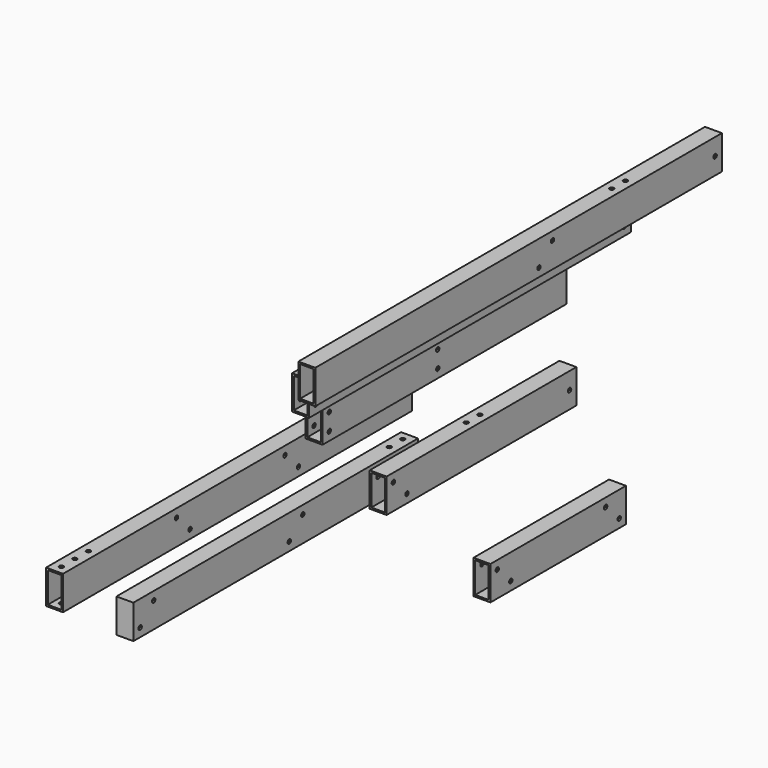
from build123d import *

# Parameters (mm, degrees)
F0_W      = 25.4
F0_H      = 50.8
F1_DEPTH  = 177.8
F2_T      = -2.54
F3_W      = 25.4
F3_H      = 50.8
F4_DEPTH  = 301.625
F5_T      = -2.54
F6_W      = 25.4
F6_H      = 50.8
F7_DEPTH  = 228.6
F8_T      = -2.54
F9_R      = 3.175
F10_DEPTH = 80.8299855063
F11_R     = 3.175
F12_DEPTH = 50.801
F13_R     = 3.175
F14_DEPTH = 63.5847636232
F15_R     = 3.175
F16_DEPTH = 223.7081707755
F17_R     = 3.175
F18_DEPTH = 25.401
F19_R     = 3.175
F20_DEPTH = 128.3850575145
F21_W     = 25.4
F21_H     = 50.8
F22_DEPTH = 381
F23_T     = -2.54
F24_R     = 3.175
F25_DEPTH = 136.5013085971
F26_R     = 3.175
F27_DEPTH = 295.0848142092
F28_W     = 25.4
F28_H     = 50.8
F29_DEPTH = 127
F30_T     = -2.54
F31_R     = 3.175
F32_DEPTH = 195.8388724098
F33_W     = 25.4
F33_H     = 50.8
F34_DEPTH = 533.4
F35_T     = -2.54
F36_W     = 25.4
F36_H     = 50.8
F37_DEPTH = 654.05
F38_T     = -2.54
F40_D     = 6.35
F40_DEPTH = 50.8
F40_TIP   = 1.9077324654
F42_D     = 6.35
F42_DEPTH = 50.8
F42_TIP   = 1.9077324654
F44_D     = 6.35
F44_DEPTH = 50.8
F44_TIP   = 1.9077324654
F47_D     = 6.35
F47_DEPTH = 50.8
F47_TIP   = 1.9077324654
F49_D     = 6.35
F49_DEPTH = 50.8
F49_TIP   = 1.9077324654
F50_D     = 6.35
F50_DEPTH = 50.8
F50_TIP   = 1.9077324654
F51_D     = 6.35
F51_DEPTH = 50.8
F51_TIP   = 1.9077324654
F52_D     = 6.35
F52_DEPTH = 50.8
F52_TIP   = 1.9077324654


# Not quite as in the source:
# - a pattern or mirror of a feature is missing from the dataset's text; its kind, count and spacing are read off the source's solid


with BuildPart() as f1:
    # F0 (on Front) → F1 (new body, symmetric)
    with BuildSketch(Plane.XZ):
        with Locations((17.2452218831, 6.8087904424)):
            Rectangle(F0_W, F0_H)
    extrude(amount=F1_DEPTH, both=True)

    # F2
    f2_openings = [f1.faces().sort_by_distance(p)[0] for p in [
        (17.245222, -177.8, 6.80879),
        (17.245222, 177.8, 6.80879),
    ]]
    offset(amount=F2_T, openings=f2_openings)

    # F9 (on face) → F10 (cut, through all)
    with BuildSketch(Plane.YZ.offset(29.9452218831)):
        with Locations((-165.1, 19.5087904424)):
            Circle(F9_R)
        with Locations((-139.7, -5.8912095576)):
            Circle(F9_R)
        with Locations((165.1, 6.8087904424)):
            Circle(F9_R)
    extrude(amount=-F10_DEPTH, mode=Mode.SUBTRACT)

    # F11 (on face) → F12 (cut, through all)
    with BuildSketch(Plane.XY.offset(32.2087904424)):
        with Locations((17.2452218831, 12.7)):
            Circle(F11_R)
        with Locations((17.2452218831, -12.7)):
            Circle(F11_R)
    extrude(amount=-F12_DEPTH, mode=Mode.SUBTRACT)


with BuildPart() as f4:
    # F3 (on Front) → F4 (new body, symmetric)
    with BuildSketch(Plane.XZ):
        with Locations((0, 179.7159612179)):
            Rectangle(F3_W, F3_H)
    extrude(amount=F4_DEPTH, both=True)

    # F5
    f5_openings = [f4.faces().sort_by_distance(p)[0] for p in [
        (0, -301.625, 179.715961),
        (0, 301.625, 179.715961),
    ]]
    offset(amount=F5_T, openings=f5_openings)

    # F13 (on face) → F14 (cut, through all)
    with BuildSketch(Plane.YZ.offset(12.7)):
        with Locations((-288.925, 192.4159612179)):
            Circle(F13_R)
        with Locations((-288.925, 167.0159612179)):
            Circle(F13_R)
    f14 = extrude(amount=-F14_DEPTH, mode=Mode.SUBTRACT)

    # F14_copies: F14 across plane
    add(f14.mirror(Plane.ZX), mode=Mode.SUBTRACT)

    # F15 (on face) → F16 (cut, through all)
    with BuildSketch(Plane.XY.offset(205.1159612179)):
        with Locations((0, -114.3)):
            Circle(F15_R)
        with Locations((0, -88.9)):
            Circle(F15_R)
    f16 = extrude(amount=-F16_DEPTH, mode=Mode.SUBTRACT)

    # F16_copies: F16 across plane
    add(f16.mirror(Plane.ZX), mode=Mode.SUBTRACT)


with BuildPart() as f7:
    # F6 (on Front) → F7 (new body, symmetric)
    with BuildSketch(Plane.XZ):
        with Locations((-38.1837636232, 102.1319037034)):
            Rectangle(F6_W, F6_H)
    extrude(amount=F7_DEPTH, both=True)

    # F8
    f8_openings = [f7.faces().sort_by_distance(p)[0] for p in [
        (-38.183764, -228.6, 102.131904),
        (-38.183764, 228.6, 102.131904),
    ]]
    offset(amount=F8_T, openings=f8_openings)

    # F17 (on face) → F18 (cut, through all)
    with BuildSketch(Plane.YZ.offset(-25.4837636232)):
        with Locations((-215.9, 114.8319037034)):
            Circle(F17_R)
        with Locations((-215.9, 89.4319037034)):
            Circle(F17_R)
        with Locations((-12.7, 114.8319037034)):
            Circle(F17_R)
        with Locations((-12.7, 89.4319037034)):
            Circle(F17_R)
    extrude(amount=-F18_DEPTH, mode=Mode.SUBTRACT)

    # F19 (on face) → F20 (cut, through all)
    with BuildSketch(Plane(origin=(0, 0, 76.7319037034), x_dir=(1, 0, 0), z_dir=(0, 0, -1))):
        with Locations((-38.1837636232, -215.9)):
            Circle(F19_R)
        with Locations((-38.1837636232, -190.5)):
            Circle(F19_R)
    extrude(amount=-F20_DEPTH, mode=Mode.SUBTRACT)


with BuildPart() as f22:
    # F21 (on Front) → F22 (new body, symmetric)
    with BuildSketch(Plane.XZ):
        with Locations((72.9165449739, 251.0926046515)):
            Rectangle(F21_W, F21_H)
    extrude(amount=F22_DEPTH, both=True)

    # F23
    f23_openings = [f22.faces().sort_by_distance(p)[0] for p in [
        (72.916545, -381, 251.092605),
        (72.916545, 381, 251.092605),
    ]]
    offset(amount=F23_T, openings=f23_openings)

    # F24 (on face) → F25 (cut, through all)
    with BuildSketch(Plane.YZ.offset(85.6165449739)):
        with Locations((368.3, 251.0926046515)):
            Circle(F24_R)
        with Locations((63.5, 263.7926046515)):
            Circle(F24_R)
        with Locations((38.1, 238.3926046515)):
            Circle(F24_R)
    extrude(amount=-F25_DEPTH, mode=Mode.SUBTRACT)

    # F26 (on face) → F27 (cut, through all)
    with BuildSketch(Plane.XY.offset(276.4926046515)):
        with Locations((72.9165449739, 215.9)):
            Circle(F26_R)
        with Locations((72.9165449739, 190.5)):
            Circle(F26_R)
    extrude(amount=-F27_DEPTH, mode=Mode.SUBTRACT)


with BuildPart() as f29:
    # F28 (on Front) → F29 (new body, symmetric)
    with BuildSketch(Plane.XZ):
        with Locations((132.2541087866, -91.8391663149)):
            Rectangle(F28_W, F28_H)
    extrude(amount=F29_DEPTH, both=True)

    # F30
    f30_openings = [f29.faces().sort_by_distance(p)[0] for p in [
        (132.254109, -127, -91.839166),
        (132.254109, 127, -91.839166),
    ]]
    offset(amount=F30_T, openings=f30_openings)

    # F31 (on face) → F32 (cut, through all)
    with BuildSketch(Plane.YZ.offset(144.9541087866)):
        with Locations((-114.3, -79.1391663149)):
            Circle(F31_R)
        with Locations((-88.9, -104.5391663149)):
            Circle(F31_R)
        with Locations((88.9, -79.1391663149)):
            Circle(F31_R)
        with Locations((114.3, -104.5391663149)):
            Circle(F31_R)
    extrude(amount=-F32_DEPTH, mode=Mode.SUBTRACT)


with BuildPart() as f34:
    # F33 (on Front) → F34 (new body)
    with BuildSketch(Plane.XZ):
        with Locations((-77.9336839914, -46.0702102427)):
            Rectangle(F33_W, F33_H)
    extrude(amount=F34_DEPTH)

    # F35
    f35_openings = [f34.faces().sort_by_distance(p)[0] for p in [
        (-77.933684, 0, -46.07021),
    ]]
    offset(amount=F35_T, openings=f35_openings)

    # F42
    with Locations(Plane(origin=(0, 0, -71.4702102427), x_dir=(1, 0, 0), z_dir=(0, 0, -1))):
        with Locations((-77.9336839914, 12.7), (-77.9336839914, 38.1)):
            Hole(F42_D / 2, depth=F42_DEPTH)
            with Locations((0, 0, -(F42_DEPTH + F42_TIP / 2))):  # 118° drill point
                Cone(0, F42_D / 2, F42_TIP, mode=Mode.SUBTRACT)

    # F47
    with Locations(Plane(origin=(-90.6336839914, 0, 0), x_dir=(0, -1, 0), z_dir=(-1, 0, 0))):
        with Locations((215.9, -33.3702102427), (241.3, -58.7702102427), (495.3, -33.3702102427), (520.7, -58.7702102427)):
            Hole(F47_D / 2, depth=F47_DEPTH)
            with Locations((0, 0, -(F47_DEPTH + F47_TIP / 2))):  # 118° drill point
                Cone(0, F47_D / 2, F47_TIP, mode=Mode.SUBTRACT)


with BuildPart() as f37:
    # F36 (on Front) → F37 (new body)
    with BuildSketch(Plane.XZ):
        with Locations((-86.9209383011, 38.1670373768)):
            Rectangle(F36_W, F36_H)
    extrude(amount=F37_DEPTH)

    # F38
    f38_openings = [f37.faces().sort_by_distance(p)[0] for p in [
        (-86.920938, 0, 38.167037),
        (-86.920938, -654.05, 38.167037),
    ]]
    offset(amount=F38_T, openings=f38_openings)

    # F40
    with Locations(Plane.XY.offset(63.5670373768)):
        with Locations((-86.9209383011, -38.1), (-86.9209383011, -12.7)):
            Hole(F40_D / 2, depth=F40_DEPTH)
            with Locations((0, 0, -(F40_DEPTH + F40_TIP / 2))):  # 118° drill point
                Cone(0, F40_D / 2, F40_TIP, mode=Mode.SUBTRACT)

    # F44
    with Locations(Plane(origin=(0, 0, 12.7670373768), x_dir=(1, 0, 0), z_dir=(0, 0, -1))):
        with Locations((-86.9209383011, 615.95), (-86.9209383011, 641.35)):
            Hole(F44_D / 2, depth=F44_DEPTH)
            with Locations((0, 0, -(F44_DEPTH + F44_TIP / 2))):  # 118° drill point
                Cone(0, F44_D / 2, F44_TIP, mode=Mode.SUBTRACT)

    # F49
    with Locations(Plane(origin=(-99.6209383011, 0, 0), x_dir=(0, -1, 0), z_dir=(-1, 0, 0))):
        with Locations((212.725, 25.4670373768)):
            Hole(F49_D / 2, depth=F49_DEPTH)
            with Locations((0, 0, -(F49_DEPTH + F49_TIP / 2))):  # 118° drill point
                Cone(0, F49_D / 2, F49_TIP, mode=Mode.SUBTRACT)

    # F50
    with Locations(Plane(origin=(-99.6209383011, 0, 0), x_dir=(0, -1, 0), z_dir=(-1, 0, 0))):
        with Locations((238.125, 50.8670373768), (441.325, 50.8670373768), (415.925, 25.4670373768)):
            Hole(F50_D / 2, depth=F50_DEPTH)
            with Locations((0, 0, -(F50_DEPTH + F50_TIP / 2))):  # 118° drill point
                Cone(0, F50_D / 2, F50_TIP, mode=Mode.SUBTRACT)

    # F51
    with Locations(Plane(origin=(0, 0, 12.7670373768), x_dir=(1, 0, 0), z_dir=(0, 0, -1))):
        with Locations((-86.9209383011, 590.55)):
            Hole(F51_D / 2, depth=F51_DEPTH)
            with Locations((0, 0, -(F51_DEPTH + F51_TIP / 2))):  # 118° drill point
                Cone(0, F51_D / 2, F51_TIP, mode=Mode.SUBTRACT)

    # F52
    with Locations(Plane(origin=(0, 0, 12.7670373768), x_dir=(1, 0, 0), z_dir=(0, 0, -1))):
        with Locations((-86.9209383011, 63.5)):
            Hole(F52_D / 2, depth=F52_DEPTH)
            with Locations((0, 0, -(F52_DEPTH + F52_TIP / 2))):  # 118° drill point
                Cone(0, F52_D / 2, F52_TIP, mode=Mode.SUBTRACT)


solid = Compound([f1.part, f4.part, f7.part, f22.part, f29.part, f34.part, f37.part])
